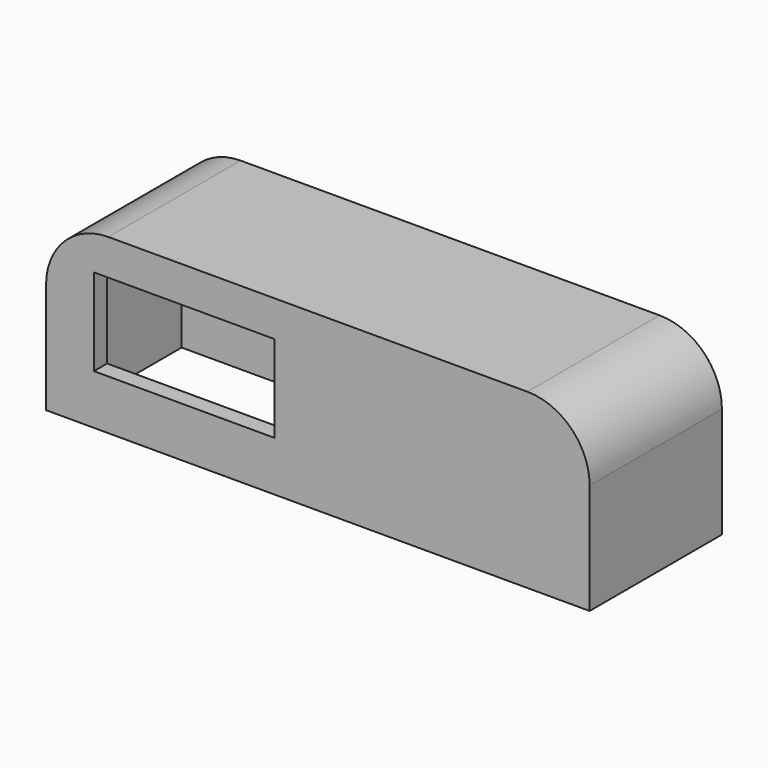
from build123d import *

# Parameters (mm, degrees)
F0_W     = 82.176
F0_H     = 26.12
F1_DEPTH = 25
F2_R     = 9.4154328933
F3_T     = -2.5
F4_W     = 27.2806887515
F4_H     = 13.1527986377
F5_DEPTH = 14.9


# Not quite as in the source:
# - a feature names something its author has since deleted; it is built from what else it names


with BuildPart() as f1:
    # F0 (on Front) → F1 (new body)
    with BuildSketch(Plane.XZ):
        with Locations((10.6781609957, 20.0886886767)):
            Rectangle(F0_W, F0_H)
    extrude(amount=F1_DEPTH)

    # F2
    f2_edges = [f1.edges().sort_by_distance(p)[0] for p in [
        (-30.409839, -12.5, 33.148689),
        (51.766161, -12.5, 33.148689),
    ]]
    fillet(f2_edges, radius=F2_R)

    # F3
    f3_openings = [f1.faces().sort_by_distance(p)[0] for p in [
        (10.678161, -12.5, 7.028689),
    ]]
    offset(amount=F3_T, openings=f3_openings)

    # F4 (on face) → F5 (cut)
    with BuildSketch(Plane.XZ.offset(25)):
        with Locations((-9.543599328, 21.1515771225)):
            Rectangle(F4_W, F4_H)
    extrude(amount=-F5_DEPTH, mode=Mode.SUBTRACT)


solid = f1.part
